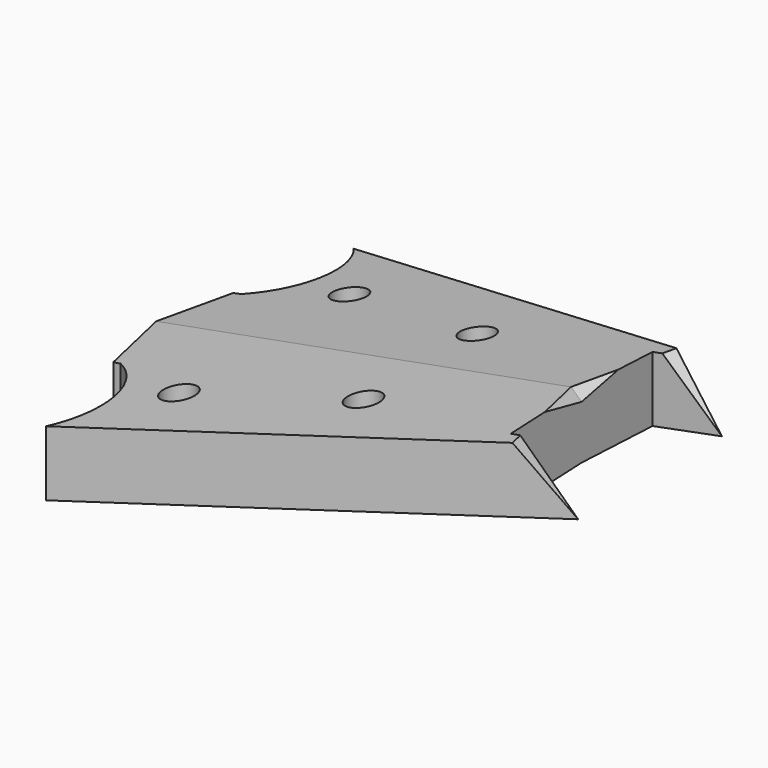
from build123d import *

# Parameters (mm, degrees)
F0_R     = 3.5
F1_DEPTH = 32.893
F3_DEPTH = 44.5826506487
F5_DEPTH = 32.894


# Not quite as in the source:
# - a feature names something its author has since deleted; it is built from what else it names


with BuildPart() as f1:
    # F0 (on Top) → F1 (new body)
    with BuildSketch(Plane.XY):
        with BuildLine():
            Line((-293, -19), (-293, 0))
            Line((-293, 0), (-394.6, 0))
            Line((-394.6, 0), (-394.6, -0.3249169361))
            ThreePointArc((-394.6, -0.3249169361), (-389.9738981677, -11.4236067086), (-378.9287209511, -16.1760579795))
            ThreePointArc((-378.9287209511, -16.1760579795), (-371.1660381492, -27.7809948386), (-374.8890577817, -41.2373289829))
            Line((-374.8890577817, -41.2373289829), (-278.3200451143, -19.2755622931))
            Line((-278.3200451143, -19.2755622931), (-293, -19))
        make_face()
        with Locations((-361.0937758916, -22.86)):
            Circle(F0_R, mode=Mode.SUBTRACT)
        with Locations((-327.5875517832, -15.24)):
            Circle(F0_R, mode=Mode.SUBTRACT)
    extrude(amount=-F1_DEPTH)

    # F2 (on face) → F3 (cut, through all)
    with BuildSketch(Plane(origin=(-9.5187600933, 41.855342378, 0), x_dir=(0.9751017202, 0.2217580556, 0), z_dir=(0.2217580556, -0.9751017202, 0))):
        Polygon((-275.6648659783, -32.893), (-275.6648659783, -14), (-374.6996750289, -32.893), align=None)
        Polygon((-374.6996750289, -18.8976), (-287.8981553787, -2.3343288283), (-275.6648659783, -14), (-275.6648659783, 0), (-374.6996750289, 0), align=None)
    extrude(amount=-F3_DEPTH, mode=Mode.SUBTRACT)

    # F4: F1 across plane


with BuildPart() as f1_1:
    add(f1.part)
    add(f1.part.mirror(Plane.XZ))

    # F5 (cut, through all): a face of the model
    f5_faces = [f1_1.faces().sort_by_distance(p)[0] for p in [
        (-387.4719249036, 0, 0),
    ]]
    extrude(f5_faces, amount=-F5_DEPTH, mode=Mode.SUBTRACT)


solid = f1_1.part
